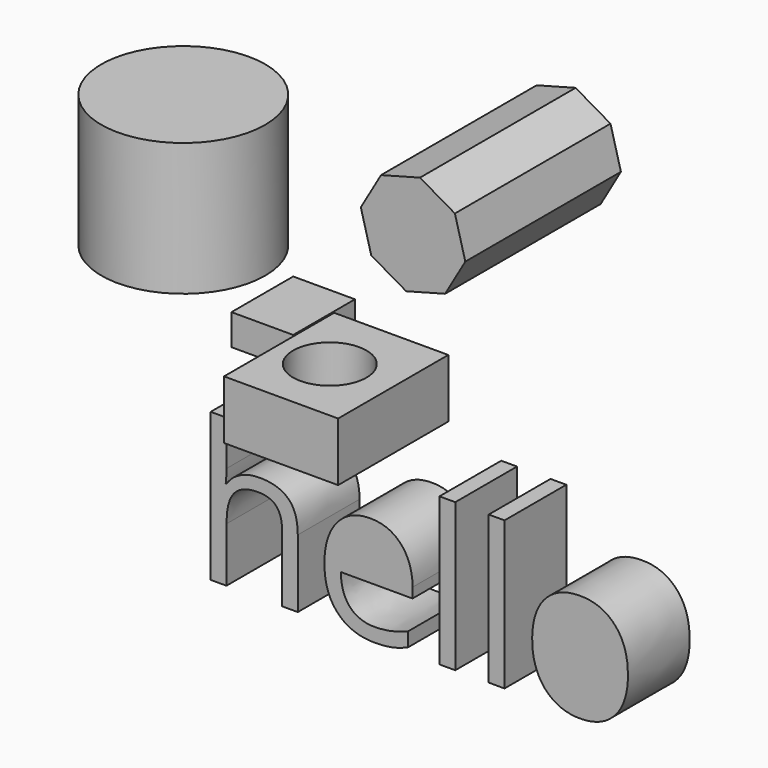
from build123d import *

# Parameters (mm, degrees)
F0_W          = 20
F0_H          = 10
F1_DEPTH      = 25
F2_R          = 26.5545261035
F3_DEPTH      = 43
F5_DEPTH      = 63
F6_W          = 36.9558222592
F6_H          = 44.5910599083
F6_R          = 11.8889080467
F7_DEPTH      = 19
F10_TEXT_SIZE = 63.0822213781
F11_DEPTH     = 25


# Not quite as in the source:
# - the program builds the solid bodies; features that only make, move or delete a surface that nothing else refers to are left out
# - Text() gives the source's letters only with a copy of the font that has no kerning and outlines rounded to 1/6400 em; it was checked with that copy


with BuildPart() as f1:
    # F0 (on Front) → F1 (new body)
    with BuildSketch(Plane.XZ):
        with Locations((10, 5)):
            Rectangle(F0_W, F0_H)
    extrude(amount=F1_DEPTH)


with BuildPart() as f3:
    # F2 (on Top) → F3 (new body)
    with BuildSketch(Plane.XY):
        with Locations((-44.3621985614, 10.9502477571)):
            Circle(F2_R)
    extrude(amount=F3_DEPTH)


with BuildPart() as f5:
    # F4 (on Front) → F5 (new body)
    with BuildSketch(Plane.XZ):
        Polygon((49.2080365472, 21.0659881273), (55.7471002288, 32.3757189176), (52.3737291655, 44.9967225246), (41.0639983752, 51.5357862063), (28.4429947682, 48.162415143), (21.9039310865, 36.8526843527), (25.2773021498, 24.2316807456), (36.5870329401, 17.692617064), align=None)
    extrude(amount=-F5_DEPTH)


with BuildPart() as f7:
    # F6 (on Top) → F7 (new body)
    with BuildSketch(Plane.XY):
        with Locations((49.7961547226, -44.858542271)):
            Rectangle(F6_W, F6_H)
        with Locations((47.9949004948, -45.1673232019)):
            Circle(F6_R, mode=Mode.SUBTRACT)
    extrude(amount=F7_DEPTH)


with BuildPart() as f11:
    # F10 (on Front) → F11 (new body)
    with BuildSketch(Plane.XZ):
        with BuildLine():
            add(Edge.make_bspline(
                [(105.2707134297, -41.8144851366), (102.7129264848, -45.1115168633), (102.7129264848, -51.6365841371)],
                knots=[0, 0, 0, 1, 1, 1], degree=2))
            add(Edge.make_bspline(
                [(102.7129264848, -51.6365841371), (102.7129264848, -58.1123684254), (105.300283221, -61.4981095259)],
                knots=[0, 0, 0, 1, 1, 1], degree=2))
            add(Edge.make_bspline(
                [(105.300283221, -61.4981095259), (107.8876399572, -64.8838506265), (112.9046478761, -64.8838506265)],
                knots=[0, 0, 0, 1, 1, 1], degree=2))
            add(Edge.make_bspline(
                [(112.9046478761, -64.8838506265), (117.9315123922, -64.8838506265), (120.5336540241, -61.5128944216)],
                knots=[0, 0, 0, 1, 1, 1], degree=2))
            add(Edge.make_bspline(
                [(120.5336540241, -61.5128944216), (123.1357956559, -58.1419382167), (123.1357956559, -51.6365841371)],
                knots=[0, 0, 0, 1, 1, 1], degree=2))
            add(Edge.make_bspline(
                [(123.1357956559, -51.6365841371), (123.1357956559, -45.2002262371), (120.5336540241, -41.8588398235)],
                knots=[0, 0, 0, 1, 1, 1], degree=2))
            add(Edge.make_bspline(
                [(120.5336540241, -41.8588398235), (117.9315123922, -38.5174534098), (112.8455082936, -38.5174534098)],
                knots=[0, 0, 0, 1, 1, 1], degree=2))
            add(Edge.make_bspline(
                [(112.8455082936, -38.5174534098), (107.8285003746, -38.5174534098), (105.2707134297, -41.8144851366)],
                knots=[0, 0, 0, 1, 1, 1], degree=2))
        make_face()
        with Locations((-12.1558560058, -68.5505047441)):
            Text('hello', F10_TEXT_SIZE, font='Open Sans', text_align=(TextAlign.LEFT, TextAlign.BOTTOM))
        with BuildLine():
            add(Edge.make_bspline(
                [(51.0200030446, -41.0308856679), (48.8663365803, -38.4583138273), (44.8547015646, -38.4583138273)],
                knots=[0, 0, 0, 1, 1, 1], degree=2))
            add(Edge.make_bspline(
                [(44.8547015646, -38.4583138273), (40.7937835634, -38.4583138273), (38.3739889777, -41.1048101461)],
                knots=[0, 0, 0, 1, 1, 1], degree=2))
            add(Edge.make_bspline(
                [(38.3739889777, -41.1048101461), (35.954194392, -43.7513064648), (35.52050412, -48.4331900827)],
                knots=[0, 0, 0, 1, 1, 1], degree=2))
            Line((35.52050412, -48.4331900827), (53.1736695088, -48.4331900827))
            add(Edge.make_bspline(
                [(53.1736695088, -48.4331900827), (53.1736695088, -43.6034575085), (51.0200030446, -41.0308856679)],
                knots=[0, 0, 0, 1, 1, 1], degree=2))
        make_face()
    extrude(amount=F11_DEPTH)


solid = Compound([f1.part, f3.part, f5.part, f7.part, f11.part])
